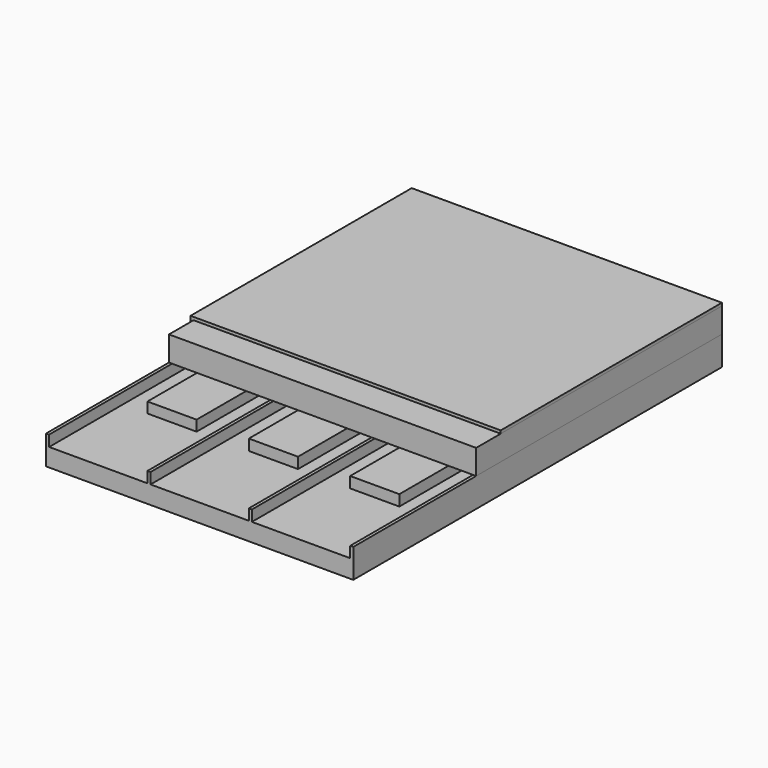
from build123d import *

# Parameters (mm, degrees)
F0_W     = 2.54
F0_H     = 9.0310877802
F1_DEPTH = 381
F0_W_2   = 40.64
F0_H_2   = 8.7648493582
F2_DEPTH = 304.8
F3_DEPTH = 254
F4_DEPTH = 228.6


with BuildPart() as f1:
    # F0 (on Front) → F1 (new body)
    with BuildSketch(Plane.XZ):
        Polygon((-153.5303335104, 7.8373091883), (-156.0703335104, 7.8373091883), (-156.0703335104, 0.3584396719), (-156.0703335104, -7.1204298445), (97.9296664896, -7.1204298445), (97.9296664896, 7.8373091883), (95.3896664896, 7.8373091883), (75.0696594866, 7.8373091883), (34.4296594866, 7.8373091883), (14.1096664896, 7.8373091883), (11.5696664896, 7.8373091883), (-8.7503335104, 7.8373091883), (-49.3903335104, 7.8373091883), (-69.7103335104, 7.8373091883), (-72.2503335104, 7.8373091883), (-92.5703335104, 7.8373091883), (-133.2103335104, 7.8373091883), align=None)
        with Locations((-154.8003335104, 12.3528530784)):
            Rectangle(F0_W, F0_H)
        with Locations((-70.9803335104, 12.3528530784)):
            Rectangle(F0_W, F0_H)
        with Locations((12.8396664896, 12.3528530784)):
            Rectangle(F0_W, F0_H)
        with Locations((96.6596664896, 12.3528530784)):
            Rectangle(F0_W, F0_H)
    extrude(amount=F1_DEPTH)


with BuildPart() as f2:
    # F0 (on Front) → F2 (new body)
    with BuildSketch(Plane.XZ):
        with Locations((-112.8903335104, 12.2197338674)):
            Rectangle(F0_W_2, F0_H_2)
    extrude(amount=F2_DEPTH)


with BuildPart() as f2b:
    # F0 (on Front) → F2, piece 2 (new body)
    with BuildSketch(Plane.XZ):
        with Locations((-29.0703335104, 12.3528530784)):
            Rectangle(F0_W_2, F0_H)
    extrude(amount=F2_DEPTH)


with BuildPart() as f2c:
    # F0 (on Front) → F2, piece 3 (new body)
    with BuildSketch(Plane.XZ):
        with Locations((54.7496594866, 12.3528530784)):
            Rectangle(F0_W_2, F0_H)
    extrude(amount=F2_DEPTH)


with BuildPart() as f3:
    # F0 (on Front) → F3 (new body)
    with BuildSketch(Plane.XZ):
        Polygon((-156.0703335104, 37.3410619795), (-156.0703335104, 16.8683969685), (-153.5303335104, 16.8683969685), (-72.2503335104, 16.8683969685), (-69.7103335104, 16.8683969685), (-49.3903335104, 16.8683969685), (-49.3903335104, 16.8913751841), (-8.7503335104, 16.8913751841), (-8.7503335104, 16.8683969685), (11.5696664896, 16.8683969685), (14.1096664896, 16.8683969685), (34.4296594866, 16.8683969685), (34.4296594866, 16.8852672009), (75.0696594866, 16.8852672009), (75.0696594866, 16.8683969685), (95.3896664896, 16.8683969685), (97.9296664896, 16.8683969685), (97.9296664896, 37.3410619795), align=None)
    extrude(amount=F3_DEPTH)


with BuildPart() as f4:
    # F0 (on Front) → F4 (new body)
    with BuildSketch(Plane.XZ):
        Polygon((-156.0703335104, 0.3584396719), (-156.0703335104, 7.8373091883), (-156.0703335104, 16.8683969685), (-156.0703335104, 37.3410619795), (97.9296664896, 37.3410619795), (97.9446843266, 39.7676415741), (-158.5593819618, 39.7676415741), (-158.5593819618, 0.3584396719), align=None)
    extrude(amount=F4_DEPTH)


solid = Compound([f1.part, f2.part, f2b.part, f2c.part, f3.part, f4.part])
